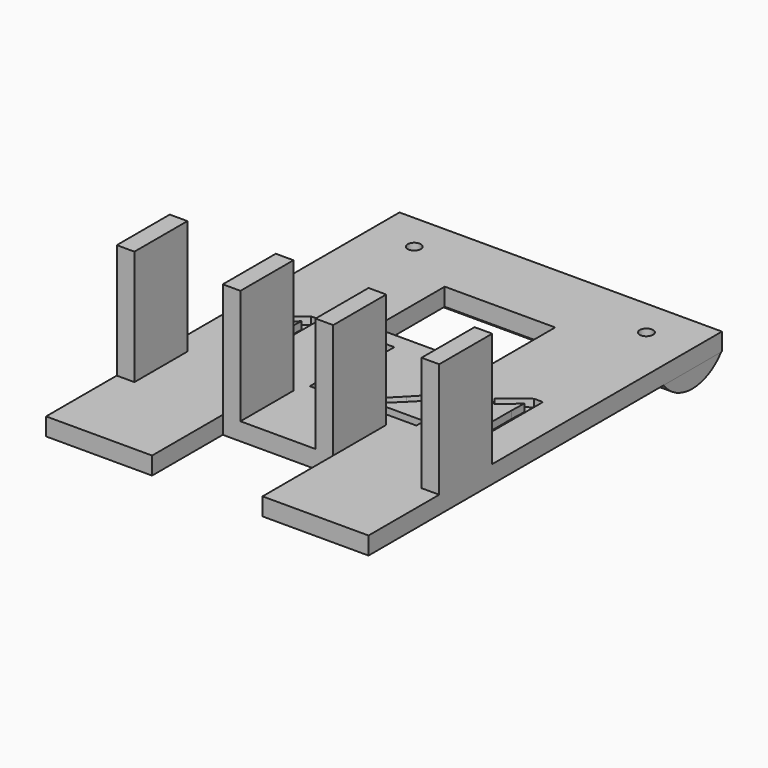
from build123d import *

# Parameters (mm, degrees)
F0_W          = 4
F0_H          = 15
F0_W_2        = 20
F0_H_2        = 20
F0_H_3        = 65
F1_DEPTH      = 4
F2_DEPTH      = 30
F5_DEPTH      = 36.5
F3_R          = 1.5
F6_DEPTH      = 8.001
F7_TEXT_SIZE  = 29.4273162985
F8_DEPTH      = 2
F8_DEPTH_BACK = 1.7


# Not quite as in the source:
# - Text() gives the source's letters only with a copy of the font that has no kerning and outlines rounded to 1/6400 em; it was checked with that copy


with BuildPart() as f1:
    # F0 (on Top) → F1 (new body)
    with BuildSketch(Plane.XY):
        with Locations((-10.5, -1.8247390879)):
            Rectangle(F0_W, F0_H)
        with Locations((-22.5, -1.8247390879)):
            Rectangle(F0_W_2, F0_H)
        with Locations((-22.5, -19.3247390879)):
            Rectangle(F0_W_2, F0_H_2)
        Polygon((-8.5, 5.6752609121), (-8.5, -9.3247390879), (0, -9.3247390879), (8.5, -9.3247390879), (8.5, 5.6752609121), (12.5, 5.6752609121), (12.5, 33.4900138964), (8.5, 33.4900138964), (0, 33.4900138964), (-8.5, 33.4900138964), (-12.5, 33.4900138964), (-12.5, 5.6752609121), align=None)
        Polygon((-32.5, 5.6752609121), (-12.5, 5.6752609121), (-12.5, 33.4900138964), (-12.5, 53.4900138964), (0, 53.4900138964), (12.5, 53.4900138964), (12.5, 33.4900138964), (12.5, 5.6752609121), (32.5, 5.6752609121), (32.5, 70.6752609121), (0, 70.6752609121), (-32.5, 70.6752609121), align=None)
        with Locations((-34.5, -1.8247390879)):
            Rectangle(F0_W, F0_H)
        with Locations((-34.5, -19.3247390879)):
            Rectangle(F0_W, F0_H_2)
        with Locations((-34.5, 38.1752609121)):
            Rectangle(F0_W, F0_H_3)
        with Locations((10.5, -1.8247390879)):
            Rectangle(F0_W, F0_H)
        with Locations((22.5, -1.8247390879)):
            Rectangle(F0_W_2, F0_H)
        with Locations((22.5, -19.3247390879)):
            Rectangle(F0_W_2, F0_H_2)
        with Locations((34.5, -1.8247390879)):
            Rectangle(F0_W, F0_H)
        with Locations((34.5, -19.3247390879)):
            Rectangle(F0_W, F0_H_2)
        with Locations((34.5, 38.1752609121)):
            Rectangle(F0_W, F0_H_3)
    extrude(amount=F1_DEPTH)

    # F0 (on Top) → F2 (join)
    with BuildSketch(Plane.XY):
        with Locations((-34.5, -1.8247390879)):
            Rectangle(F0_W, F0_H)
        with Locations((-10.5, -1.8247390879)):
            Rectangle(F0_W, F0_H)
        with Locations((10.5, -1.8247390879)):
            Rectangle(F0_W, F0_H)
        with Locations((34.5, -1.8247390879)):
            Rectangle(F0_W, F0_H)
    extrude(amount=F2_DEPTH)


with BuildPart() as f5:
    # F4 (on Right) → F5 (new body, symmetric)
    with BuildSketch(Plane.YZ):
        with BuildLine():
            Line((62.2996781021, 0), (54.1295077664, 0))
            ThreePointArc((54.1295077664, 0), (57.751280491, -2.946335395), (62.2996781021, -4))
            Line((62.2996781021, -4), (62.2996781021, 0))
        make_face()
        with BuildLine():
            Line((62.2996781021, 0), (62.2996781021, -4))
            ThreePointArc((62.2996781021, -4), (66.8480757133, -2.946335395), (70.4698484379, 0))
            Line((70.4698484379, 0), (62.2996781021, 0))
        make_face()
    extrude(amount=F5_DEPTH, both=True)


with BuildPart() as f6_tool:
    # F3 (on face) → F6 (new body, through all)
    with BuildSketch(Plane.XY.offset(4)):
        with BuildLine():
            ThreePointArc((27.777596131, 62.0826374043), (26.277596131, 63.5826374043), (24.777596131, 62.0826374043))
            ThreePointArc((24.777596131, 62.0826374043), (26.277596131, 60.5826374043), (27.777596131, 62.0826374043))
        make_face()
        with Locations((-26.277596131, 62.0826374043)):
            Circle(F3_R)
    extrude(amount=-F6_DEPTH)


with BuildPart() as f1_1:
    add(f1.part)

    # F6: cut by f6_tool
    add(f6_tool.part, mode=Mode.SUBTRACT)

    # F7 (on face) → F8 (cut, two sides)
    with BuildSketch(Plane.XY.offset(4)) as f8_sk:
        with Locations((-32.0872962475, 8.8290246204)):
            Text('1121', F7_TEXT_SIZE, font='Open Sans', text_align=(TextAlign.LEFT, TextAlign.BOTTOM))
    extrude(amount=F8_DEPTH, mode=Mode.SUBTRACT)
    extrude(f8_sk.sketch, amount=-F8_DEPTH_BACK, mode=Mode.SUBTRACT)


with BuildPart() as f5_1:
    add(f5.part)

    # F6: cut by f6_tool
    add(f6_tool.part, mode=Mode.SUBTRACT)


solid = Compound([f1_1.part, f5_1.part])
